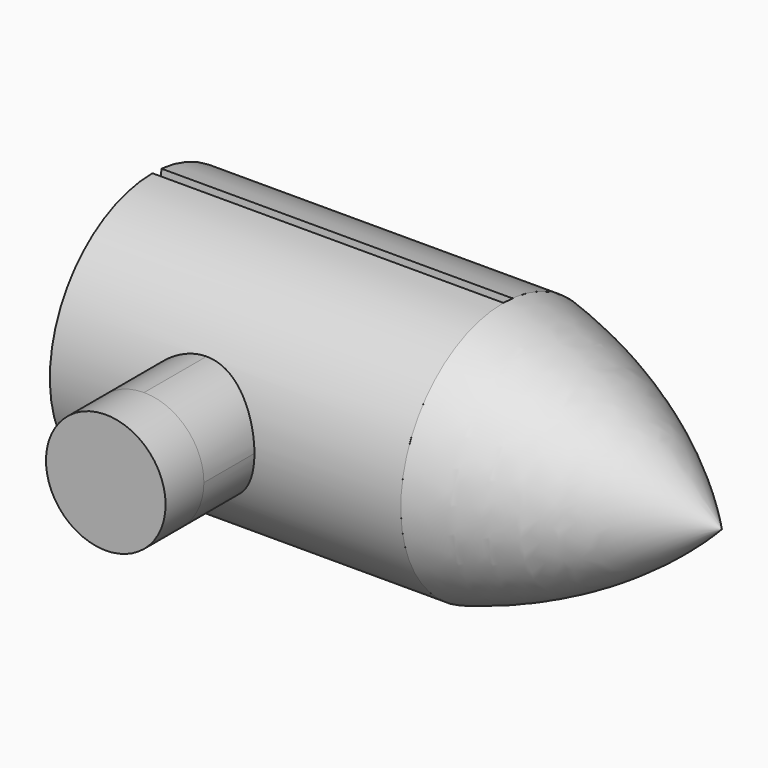
from build123d import *
from build123d import SkipClean  # not in build123d's __all__

# Parameters (mm, degrees)
F0_W     = 46.5685683415
F0_H     = 17.018
F1_ANGLE = 355
F3_D     = 28.829
F3_DEPTH = 50.8
F3_TIP   = 8.661105393
F8_R     = 7.9375
F9_DEPTH = 6.35


with BuildPart() as f1:
    # F0 (on Front) → F1 (revolve)
    with BuildSketch(Plane.XZ):
        with Locations((-63.3321542538, 22.987)):
            Rectangle(F0_W, F0_H)
    revolve(axis=Axis((-48.8339384246, 0, 14.478), (1, 0, 0)), revolution_arc=F1_ANGLE)

    # F3
    with Locations(Plane(origin=(-86.6164384246, 0, 0), x_dir=(0, -1, 0), z_dir=(-1, 0, 0))):
        with Locations((0, 14.478)):
            Hole(F3_D / 2, depth=F3_DEPTH)
            with Locations((0, 0, -(F3_DEPTH + F3_TIP / 2))):  # 118° drill point
                Cone(0, F3_D / 2, F3_TIP, mode=Mode.SUBTRACT)

    # F6 (on offset) → F7 (join, up to the next surface of F1)
    with BuildSketch(Plane.XZ.offset(25.4)):
        with BuildLine():
            Line((-67.4114227295, 14.5107703283), (-59.4739227295, 14.5107703283))
            ThreePointArc((-59.4739227295, 14.5107703283), (-61.7987626538, 20.123430404), (-67.4114227295, 22.4482703283))
            Line((-67.4114227295, 22.4482703283), (-67.4114227295, 14.5107703283))
        make_face()
        with BuildLine():
            ThreePointArc((-67.4114227295, 22.4482703283), (-73.0240828052, 8.8981102527), (-59.4739227295, 14.5107703283))
            Line((-59.4739227295, 14.5107703283), (-67.4114227295, 14.5107703283))
            Line((-67.4114227295, 14.5107703283), (-67.4114227295, 22.4482703283))
        make_face()
    extrude(until=Until.NEXT, dir=(0, 1, 0))

    # F8 (on face) → F9 (join)
    with BuildSketch(Plane.XZ.offset(25.4)):
        with Locations((-67.4114227295, 14.5107703283)):
            Circle(F8_R)
    with SkipClean():  # cleaning this boolean's faces spoils the solid; the shape is the same uncleaned
        extrude(amount=F9_DEPTH)


with BuildPart() as f4:
    # F0 (on Front) → F4 (revolve)
    with BuildSketch(Plane.XZ):
        with BuildLine():
            ThreePointArc((-11.0514384246, 14.478), (-24.3874453928, 24.9672508998), (-40.0478700831, 31.496))
            Line((-40.0478700831, 31.496), (-40.0478700831, 14.478))
            Line((-40.0478700831, 14.478), (-11.0514384246, 14.478))
        make_face()
    revolve(axis=Axis((-48.8339384246, 0, 14.478), (1, 0, 0)))


solid = Compound([f1.part, f4.part])
